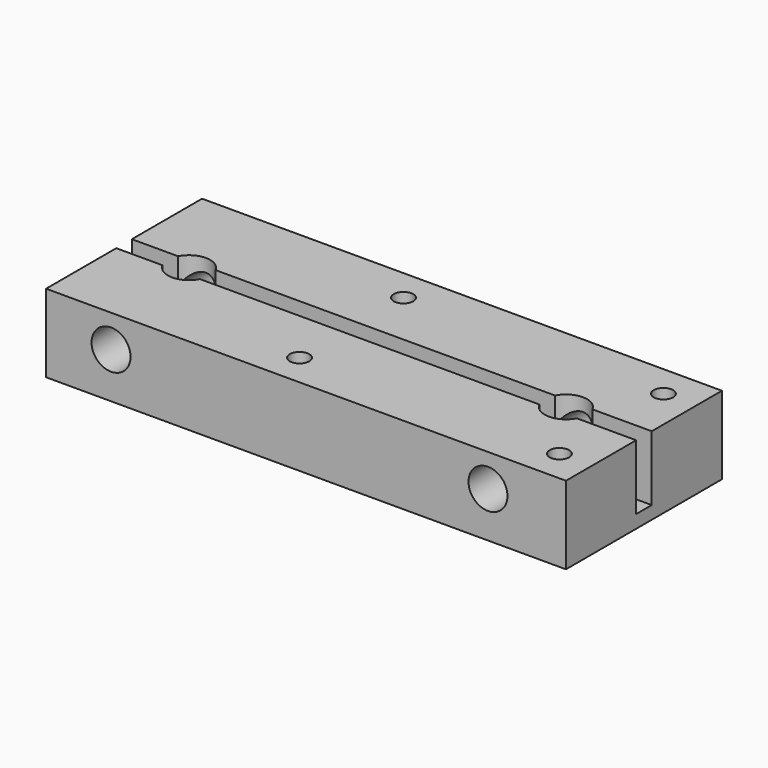
from build123d import *

# Parameters (mm, degrees)
F0_W     = 80
F0_H     = 30
F1_DEPTH = 12
F2_R     = 1.5
F3_DEPTH = 25
F5_DEPTH = 5
F6_DEPTH = 10
F7_R     = 3
F8_DEPTH = 30.001


with BuildPart() as f1:
    # F0 (on Top) → F1 (new body)
    with BuildSketch(Plane.XY):
        with Locations((40, 15)):
            Rectangle(F0_W, F0_H)
    extrude(amount=F1_DEPTH)

    # F2 (on face) → F3 (cut)
    with BuildSketch(Plane.XY.offset(12)):
        with Locations((35, 5)):
            Circle(F2_R)
        with Locations((35, 25)):
            Circle(F2_R)
        with Locations((75, 5)):
            Circle(F2_R)
        with Locations((75, 25)):
            Circle(F2_R)
    extrude(amount=-F3_DEPTH, mode=Mode.SUBTRACT)

    # F4 (on face) → F5 (cut)
    with BuildSketch(Plane.XY.offset(12)):
        with BuildLine():
            Line((42.8169872981, 13.5), (65.1168593513, 13.5))
            ThreePointArc((65.1168593513, 13.5), (68, 11.75), (70.8831406487, 13.5))
            Line((70.8831406487, 13.5), (80, 13.5))
            Line((80, 13.5), (80, 16.5))
            Line((80, 16.5), (70.8831406487, 16.5))
            ThreePointArc((70.8831406487, 16.5), (68, 18.25), (65.1168593513, 16.5))
            Line((65.1168593513, 16.5), (42.8169872981, 16.5))
            Line((42.8169872981, 16.5), (12.8831406487, 16.5))
            ThreePointArc((12.8831406487, 16.5), (10, 18.25), (7.1168593513, 16.5))
            Line((7.1168593513, 16.5), (0, 16.5))
            Line((0, 16.5), (0, 13.5))
            Line((0, 13.5), (7.1168593513, 13.5))
            ThreePointArc((7.1168593513, 13.5), (10, 11.75), (12.8831406487, 13.5))
            Line((12.8831406487, 13.5), (42.8169872981, 13.5))
        make_face()
    extrude(amount=-F5_DEPTH, mode=Mode.SUBTRACT)

    # F4 (on face) → F6 (cut)
    with BuildSketch(Plane.XY.offset(12)):
        with BuildLine():
            Line((42.8169872981, 13.5), (65.1168593513, 13.5))
            ThreePointArc((65.1168593513, 13.5), (68, 11.75), (70.8831406487, 13.5))
            Line((70.8831406487, 13.5), (80, 13.5))
            Line((80, 13.5), (80, 16.5))
            Line((80, 16.5), (70.8831406487, 16.5))
            ThreePointArc((70.8831406487, 16.5), (68, 18.25), (65.1168593513, 16.5))
            Line((65.1168593513, 16.5), (42.8169872981, 16.5))
            Line((42.8169872981, 16.5), (12.8831406487, 16.5))
            ThreePointArc((12.8831406487, 16.5), (10, 18.25), (7.1168593513, 16.5))
            Line((7.1168593513, 16.5), (0, 16.5))
            Line((0, 16.5), (0, 13.5))
            Line((0, 13.5), (7.1168593513, 13.5))
            ThreePointArc((7.1168593513, 13.5), (10, 11.75), (12.8831406487, 13.5))
            Line((12.8831406487, 13.5), (42.8169872981, 13.5))
        make_face()
    extrude(amount=-F6_DEPTH, mode=Mode.SUBTRACT)

    # F7 (on face) → F8 (cut, through all)
    with BuildSketch(Plane(origin=(0, 30, 0), x_dir=(-1, 0, 0), z_dir=(0, 1, 0))):
        with Locations((-68, 7)):
            Circle(F7_R)
        with Locations((-10, 7)):
            Circle(F7_R)
    extrude(amount=-F8_DEPTH, mode=Mode.SUBTRACT)


solid = f1.part
